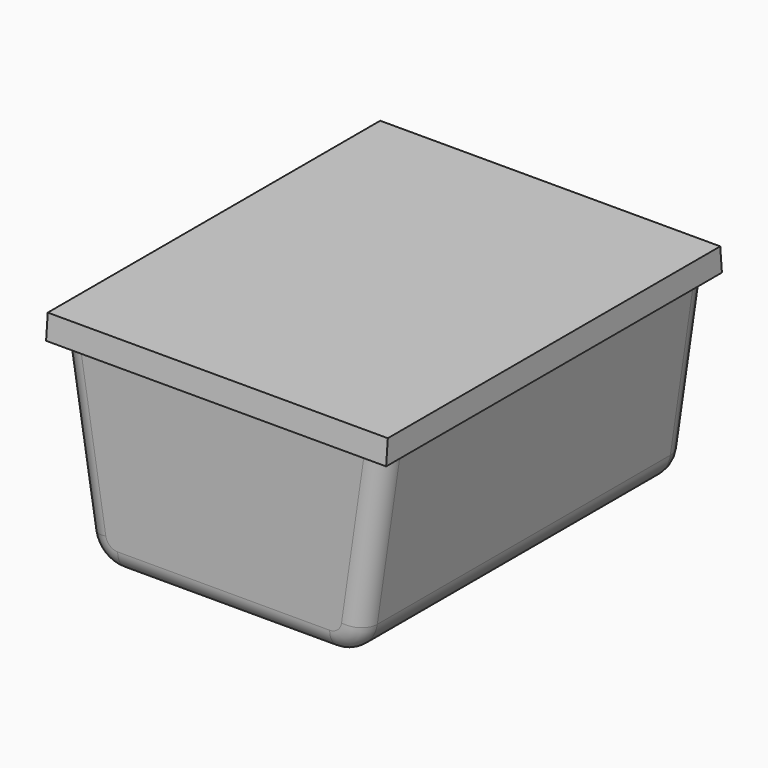
from build123d import *

# Parameters (mm, degrees)
F1_DEPTH     = 101.22
F3_DEPTH     = 3
F5_DEPTH     = 3
F6_T1_DEPTH  = 52.0304782215
F6_T3_DEPTH  = 53.0410614462
F6_T5_DEPTH  = 52.232484609
F6_T8_ANGLE  = 81.7241071729
F6_T10_ANGLE = 80.9097230792
F7_R         = 5
F9_DEPTH     = 6
F11_DEPTH    = 111.14


# Not quite as in the source:
# - a fillet or chamfer that OpenCascade refuses, or shapes differently, is made with other operations: its cross-section is extruded or revolved along the edge and cut away or added


with BuildPart() as f1:
    # F0 (on Front) → F1 (new body)
    with BuildSketch(Plane.XZ):
        with BuildLine():
            Line((57.3046570067, 0), (4.2635955605, 0))
            ThreePointArc((4.2635955605, 0), (1.0193516214, 1.1954131284), (-0.6736075991, 4.2100474945))
            Line((-0.6736075991, 4.2100474945), (-7.04, 44))
            Line((-7.04, 44), (-10.0781573363, 44))
            Line((-10.0781573363, 44), (-3.6359294949, 3.7360759911))
            ThreePointArc((-3.6359294949, 3.7360759911), (-0.927194742, -1.0873389946), (4.2635955605, -3))
            Line((4.2635955605, -3), (57.3046570067, -3))
            ThreePointArc((57.3046570067, -3), (62.5385776153, -1.0502954525), (65.221348521, 3.8484812343))
            Line((65.221348521, 3.8484812343), (71.0615694323, 44))
            Line((71.0615694323, 44), (68.03, 44))
            Line((68.03, 44), (62.2525892031, 4.2803007714))
            ThreePointArc((62.2525892031, 4.2803007714), (60.5758573871, 1.2185653422), (57.3046570067, 0))
        make_face()
    extrude(amount=F1_DEPTH)

    # F2 (on face) → F3 (join)
    with BuildSketch(Plane.XZ.offset(101.22)):
        with BuildLine():
            Line((68.03, 44), (-7.04, 44))
            Line((-7.04, 44), (-0.6736075991, 4.2100474945))
            ThreePointArc((-0.6736075991, 4.2100474945), (1.0193516214, 1.1954131284), (4.2635955605, 0))
            Line((4.2635955605, 0), (57.3046570067, 0))
            ThreePointArc((57.3046570067, 0), (60.5758573871, 1.2185653422), (62.2525892031, 4.2803007714))
            Line((62.2525892031, 4.2803007714), (68.03, 44))
        make_face()
    extrude(amount=-F3_DEPTH)

    # F6: fillet of radius 5 on 1 edges, made by hand

    # F6_s2 → F6_t1 (cut)
    with BuildSketch(Plane(origin=(1.8994814012, 0, 13.0589346335), x_dir=(0, 1, 0), z_dir=(0.1439398457, 0, 0.9895864393))):
        with BuildLine():
            ThreePointArc((-4.582575695, -63.9882122531), (-1.8439629074, -63.1715123858), (0, -60.9882122531))
            Line((0, -60.9882122531), (0, -63.9882122531))
            Line((0, -63.9882122531), (-4.582575695, -63.9882122531))
        make_face()
    extrude(amount=F6_T1_DEPTH, mode=Mode.SUBTRACT)

    # F6_s4 → F6_t3 (cut)
    with BuildSketch(Plane.YZ.offset(4.2635955605)):
        with BuildLine():
            ThreePointArc((-4.582575695, -3), (-1.8439629074, -2.1833001327), (0, 0))
            Line((0, 0), (0, -3))
            Line((0, -3), (-4.582575695, -3))
        make_face()
    extrude(amount=F6_T3_DEPTH, mode=Mode.SUBTRACT)

    # F6_s6 → F6_t5 (cut)
    with BuildSketch(Plane(origin=(-8.9258440165, 0, 55.7865251034), x_dir=(0, 1, 0), z_dir=(0.1579905011, 0, -0.9874406319))):
        with BuildLine():
            ThreePointArc((-4.582575695, -3), (-1.8439629074, -2.1833001327), (0, 0))
            Line((0, 0), (0, -3))
            Line((0, -3), (-4.582575695, -3))
        make_face()
    extrude(amount=F6_T5_DEPTH, mode=Mode.SUBTRACT)

    # F6_s7 → F6_t8 (revolve, cut)
    with BuildSketch(Plane.YZ.offset(57.3046570067)):
        with BuildLine():
            ThreePointArc((0, 0), (-1.8439629074, -2.1833001327), (-4.582575695, -3))
            Line((-4.582575695, -3), (0, -3))
            Line((0, -3), (0, 0))
        make_face()
    revolve(axis=Axis((57.3046570067, 0, 5), (0, -1, 0)), revolution_arc=F6_T8_ANGLE, mode=Mode.SUBTRACT)

    # F6_s9 → F6_t10 (revolve, cut)
    with BuildSketch(Plane(origin=(-0.6736075991, 0, 4.2100474945), x_dir=(0, 1, 0), z_dir=(-0.1579905011, 0, 0.9874406319))):
        with BuildLine():
            ThreePointArc((-4.582575695, 3), (-1.8439629074, 2.1833001327), (0, 0))
            Line((0, 0), (0, 3))
            Line((0, 3), (-4.582575695, 3))
        make_face()
    revolve(axis=Axis((4.2635955605, 0, 5), (0, -1, 0)), revolution_arc=F6_T10_ANGLE, mode=Mode.SUBTRACT)

    # F7
    f7_edges = [f1.edges().sort_by_distance(p)[0] for p in [
        (-6.857043, -101.22, 23.868038),
        (68.141459, -101.22, 23.924241),
        (-0.927195, -101.22, -1.087339),
        (30.784126, -101.22, -3),
        (62.538578, -101.22, -1.050295),
    ]]
    fillet(f7_edges, radius=F7_R)


with BuildPart() as f5:
    # F4 (on face) → F5 (new body)
    with BuildSketch(Plane(origin=(0, 0, 0), x_dir=(-1, 0, 0), z_dir=(0, 1, 0))):
        with BuildLine():
            ThreePointArc((-4.2635955605, 0), (-1.0193516214, 1.1954131284), (0.6736075991, 4.2100474945))
            Line((0.6736075991, 4.2100474945), (7.04, 44))
            Line((7.04, 44), (-68.03, 44))
            Line((-68.03, 44), (-62.2525892031, 4.2803007714))
            ThreePointArc((-62.2525892031, 4.2803007714), (-60.5758573871, 1.2185653422), (-57.3046570067, 0))
            Line((-57.3046570067, 0), (-4.2635955605, 0))
        make_face()
    extrude(amount=-F5_DEPTH)


with BuildPart() as f9:
    # F8 (on face) → F9 (new body)
    with BuildSketch(Plane.XY.offset(44)):
        Polygon((-12.04, 1.78), (-12.04, -98.22), (-12.04, -103.22), (73.03, -103.22), (73.03, -98.22), (73.03, -3.22), (73.03, 1.78), align=None)
    extrude(amount=F9_DEPTH)

    # F10 (on face) → F11 (cut)
    with BuildSketch(Plane(origin=(-12.04, 0, 0), x_dir=(0, -1, 0), z_dir=(-1, 0, 0))):
        Polygon((102.6950680188, 50), (103.22, 44), (103.22, 50), align=None)
        Polygon((-1.78, 50), (-1.78, 44), (-1.2550680188, 50), align=None)
    extrude(amount=-F11_DEPTH, mode=Mode.SUBTRACT)


solid = Compound([f1.part, f5.part, f9.part])
